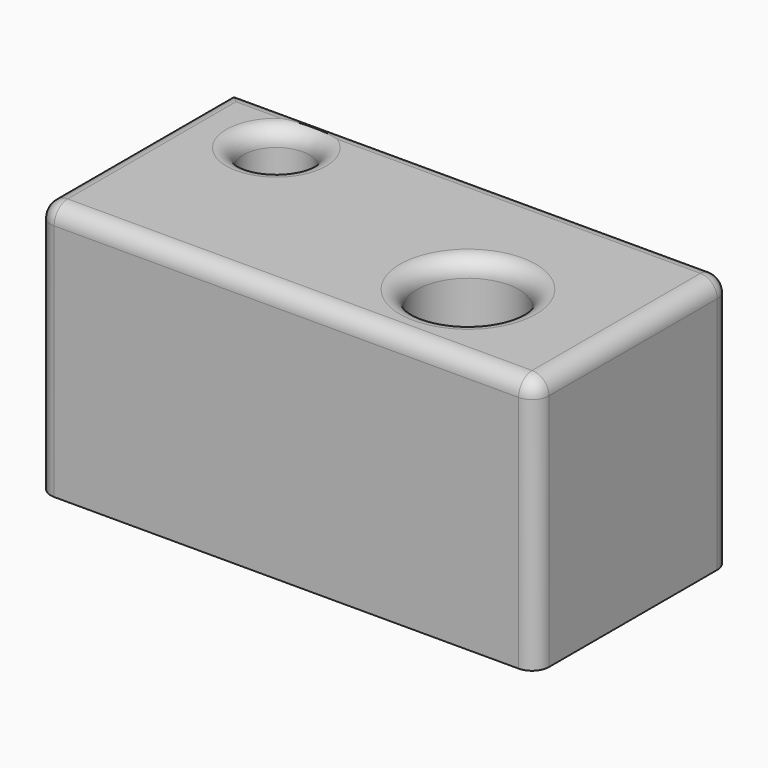
from build123d import *

# Parameters (mm, degrees)
F0_W         = 150
F0_H         = 73.4827055006
F0_R         = 15.3666463422
F0_R_2       = 9.9309311283
F1_DEPTH     = 76.962
F2_T1_DEPTH  = 139.84
F2_T3_DEPTH  = 63.3227055006
F2_T5_DEPTH  = 157.62
F2_T7_DEPTH  = 81.1027055006
F2_T9_DEPTH  = 84.582
F2_S13_W     = 5.08
F2_S13_H     = 5.08
F2_T14_DEPTH = 5.08
F2_S19_W     = 5.08
F2_S19_H     = 5.08
F2_T20_DEPTH = 5.08
F2_S25_W     = 5.08
F2_S25_H     = 5.08
F2_T26_DEPTH = 5.08


# Not quite as in the source:
# - a fillet or chamfer that OpenCascade refuses, or shapes differently, is made with other operations: its cross-section is extruded or revolved along the edge and cut away or added


with BuildPart() as f1:
    # F0 (on Top) → F1 (new body)
    with BuildSketch(Plane.XY):
        with Locations((19.2005559802, -34.1252638027)):
            Rectangle(F0_W, F0_H)
        with Locations((51.502276212, -42.9059304297)):
            Circle(F0_R, mode=Mode.SUBTRACT)
        with Locations((-28.6887511611, -14.8067288101)):
            Circle(F0_R_2, mode=Mode.SUBTRACT)
    extrude(amount=F1_DEPTH)

    # F2: fillet of radius 5.08 on 9 edges, made by hand

    # F2_s2 → F2_t1 (cut)
    with BuildSketch(Plane.YZ.offset(-50.7194440198)):
        with BuildLine():
            ThreePointArc((-70.866616553, 71.882), (-69.3787190014, 75.4741024484), (-65.786616553, 76.962))
            Line((-65.786616553, 76.962), (-70.866616553, 76.962))
            Line((-70.866616553, 76.962), (-70.866616553, 71.882))
        make_face()
    extrude(amount=F2_T1_DEPTH, mode=Mode.SUBTRACT)

    # F2_s4 → F2_t3 (cut)
    with BuildSketch(Plane.XZ.offset(2.4639110524)):
        with BuildLine():
            ThreePointArc((94.2005559802, 71.882), (92.7126584286, 75.4741024484), (89.1205559802, 76.962))
            Line((89.1205559802, 76.962), (94.2005559802, 76.962))
            Line((94.2005559802, 76.962), (94.2005559802, 71.882))
        make_face()
    extrude(amount=F2_T3_DEPTH, mode=Mode.SUBTRACT)

    # F2_s6 → F2_t5 (cut)
    with BuildSketch(Plane.YZ.offset(-68.4994440198)):
        with BuildLine():
            ThreePointArc((2.6160889476, 71.882), (1.128191396, 75.4741024484), (-2.4639110524, 76.962))
            Line((-2.4639110524, 76.962), (2.6160889476, 76.962))
            Line((2.6160889476, 76.962), (2.6160889476, 71.882))
        make_face()
    extrude(amount=F2_T5_DEPTH, mode=Mode.SUBTRACT)

    # F2_s8 → F2_t7 (cut)
    with BuildSketch(Plane.XZ.offset(-15.3160889476)):
        with BuildLine():
            ThreePointArc((-55.7994440198, 71.882), (-54.3115464682, 75.4741024484), (-50.7194440198, 76.962))
            Line((-50.7194440198, 76.962), (-55.7994440198, 76.962))
            Line((-55.7994440198, 76.962), (-55.7994440198, 71.882))
        make_face()
    extrude(amount=F2_T7_DEPTH, mode=Mode.SUBTRACT)

    # F2_s10 → F2_t9 (cut)
    with BuildSketch(Plane.XY.offset(-12.7)):
        with BuildLine():
            ThreePointArc((89.1205559802, -70.866616553), (92.7126584286, -69.3787190014), (94.2005559802, -65.786616553))
            Line((94.2005559802, -65.786616553), (94.2005559802, -70.866616553))
            Line((94.2005559802, -70.866616553), (89.1205559802, -70.866616553))
        make_face()
        with BuildLine():
            ThreePointArc((89.1205559802, 2.6160889476), (92.7126584286, 1.128191396), (94.2005559802, -2.4639110524))
            Line((94.2005559802, -2.4639110524), (94.2005559802, 2.6160889476))
            Line((94.2005559802, 2.6160889476), (89.1205559802, 2.6160889476))
        make_face()
        with BuildLine():
            ThreePointArc((-55.7994440198, -65.786616553), (-54.3115464682, -69.3787190014), (-50.7194440198, -70.866616553))
            Line((-50.7194440198, -70.866616553), (-55.7994440198, -70.866616553))
            Line((-55.7994440198, -70.866616553), (-55.7994440198, -65.786616553))
        make_face()
    extrude(amount=F2_T9_DEPTH, mode=Mode.SUBTRACT)


with BuildPart() as f2_tool12:
    # F2_s13 → F2_t14 (new body)
    with BuildSketch(Plane.YZ.offset(-50.7194440198)):
        with Locations((-68.326616553, 74.422)):
            Rectangle(F2_S13_W, F2_S13_H)
    extrude(amount=-F2_T14_DEPTH)

    # F2_s15 → F2_t16 (revolve, cut)
    with BuildSketch(Plane(origin=(-50.7194440198, -65.786616553, 71.882), x_dir=(0, 0.7071067812, -0.7071067812), z_dir=(0, 0.7071067812, 0.7071067812))):
        with BuildLine():
            ThreePointArc((0, -5.08), (5.08, 0), (0, 5.08))
            Line((0, 5.08), (0, -5.08))
        make_face()
    revolve(axis=Axis((-50.7194440198, -65.786616553, 71.882), (-1, 0, 0)), mode=Mode.SUBTRACT)


with BuildPart() as f1_1:
    add(f1.part)

    # F2_t11: cut F2_tool12
    add(f2_tool12.part, mode=Mode.SUBTRACT)


with BuildPart() as f2_tool18:
    # F2_s19 → F2_t20 (new body)
    with BuildSketch(Plane.XZ.offset(65.786616553)):
        with Locations((91.6605559802, 74.422)):
            Rectangle(F2_S19_W, F2_S19_H)
    extrude(amount=F2_T20_DEPTH)

    # F2_s21 → F2_t22 (revolve, cut)
    with BuildSketch(Plane(origin=(89.1205559802, -65.786616553, 71.882), x_dir=(-0.7071067812, 0, -0.7071067812), z_dir=(-0.7071067812, 0, 0.7071067812))):
        with BuildLine():
            ThreePointArc((0, -5.08), (5.08, 0), (0, 5.08))
            Line((0, 5.08), (0, -5.08))
        make_face()
    revolve(axis=Axis((89.1205559802, -65.786616553, 71.882), (0, -1, 0)), mode=Mode.SUBTRACT)


with BuildPart() as f1_2:
    add(f1_1.part)

    # F2_t17: cut F2_tool18
    add(f2_tool18.part, mode=Mode.SUBTRACT)


with BuildPart() as f2_tool24:
    # F2_s25 → F2_t26 (new body)
    with BuildSketch(Plane.XZ.offset(2.4639110524)):
        with Locations((91.6605559802, 74.422)):
            Rectangle(F2_S25_W, F2_S25_H)
    extrude(amount=-F2_T26_DEPTH)

    # F2_s27 → F2_t28 (revolve, cut)
    with BuildSketch(Plane(origin=(89.1205559802, -2.4639110524, 71.882), x_dir=(-0.7071067812, 0, -0.7071067812), z_dir=(0.7071067812, 0, -0.7071067812))):
        with BuildLine():
            ThreePointArc((0, -5.08), (5.08, 0), (0, 5.08))
            Line((0, 5.08), (0, -5.08))
        make_face()
    revolve(axis=Axis((89.1205559802, -2.4639110524, 71.882), (0, 1, 0)), mode=Mode.SUBTRACT)


with BuildPart() as f1_3:
    add(f1_2.part)

    # F2_t23: cut F2_tool24
    add(f2_tool24.part, mode=Mode.SUBTRACT)

    # F2_s29 → F2_t30 (revolve, cut)
    with BuildSketch(Plane.XZ.offset(42.9059304297)):
        with BuildLine():
            ThreePointArc((66.8689225542, 71.882), (68.3568201058, 75.4741024484), (71.9489225542, 76.962))
            Line((71.9489225542, 76.962), (66.8689225542, 76.962))
            Line((66.8689225542, 76.962), (66.8689225542, 71.882))
        make_face()
    revolve(axis=Axis((51.502276212, -42.9059304297, 76.962), (0, 0, 1)), mode=Mode.SUBTRACT)

    # F2_s31 → F2_t32 (revolve, cut)
    with BuildSketch(Plane.XZ.offset(14.8067288101)):
        with BuildLine():
            ThreePointArc((-18.7578200328, 71.882), (-17.2699224813, 75.4741024484), (-13.6778200328, 76.962))
            Line((-13.6778200328, 76.962), (-18.7578200328, 76.962))
            Line((-18.7578200328, 76.962), (-18.7578200328, 71.882))
        make_face()
    revolve(axis=Axis((-28.6887511611, -14.8067288101, 76.962), (0, 0, 1)), mode=Mode.SUBTRACT)


solid = f1_3.part
